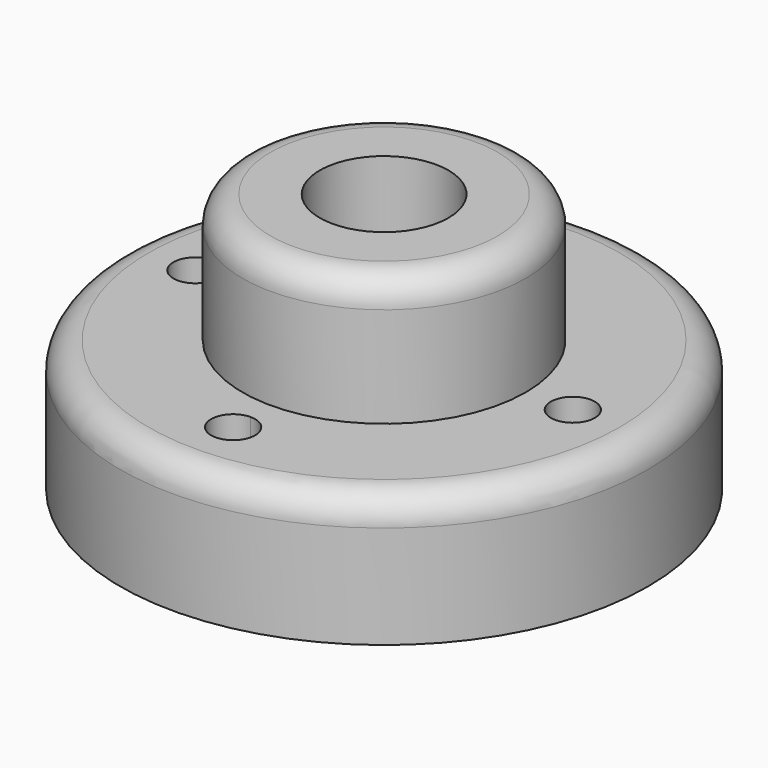
from build123d import *

# Parameters (mm, degrees)
F0_R     = 30
F0_R_2   = 16.1
F1_DEPTH = 14.9
F2_DEPTH = 29.5
F3_R     = 3.2
F4_R     = 3.2
F5_R     = 2.5
F6_DEPTH = 100
F7_R     = 7.315
F8_DEPTH = 100


with BuildPart() as f1:
    # F0 (on Top) → F1 (new body)
    with BuildSketch(Plane.XY):
        Circle(F0_R)
        Circle(F0_R_2, mode=Mode.SUBTRACT)
    extrude(amount=F1_DEPTH)

    # F0 (on Top) → F2 (join)
    with BuildSketch(Plane.XY):
        Circle(F0_R_2)
    extrude(amount=F2_DEPTH)

    # F3
    f3_edges = [f1.edges().sort_by_distance(p)[0] for p in [
        (-30, 0, 14.9),
    ]]
    fillet(f3_edges, radius=F3_R)

    # F4
    f4_edges = [f1.edges().sort_by_distance(p)[0] for p in [
        (-16.1, 0, 29.5),
    ]]
    fillet(f4_edges, radius=F4_R)

    # F5 (on face) → F6 (cut)
    with BuildSketch(Plane.XY.offset(14.9)):
        with Locations((0, 21.45)):
            Circle(F5_R)
        with BuildLine():
            ThreePointArc((23.95, 0), (21.45, 2.5), (18.95, 0))
            ThreePointArc((18.95, 0), (21.45, -2.5), (23.95, 0))
        make_face()
        with BuildLine():
            ThreePointArc((2.5, -21.45), (1.767766953, -19.682233047), (0, -18.95))
            ThreePointArc((0, -18.95), (-2.5, -21.45), (0, -23.95))
            ThreePointArc((0, -23.95), (1.767766953, -23.217766953), (2.5, -21.45))
        make_face()
        with Locations((-21.45, 0)):
            Circle(F5_R)
    extrude(amount=-F6_DEPTH, mode=Mode.SUBTRACT)

    # F7 (on face) → F8 (cut)
    with BuildSketch(Plane.XY.offset(29.5)):
        Circle(F7_R)
    extrude(amount=-F8_DEPTH, mode=Mode.SUBTRACT)


solid = f1.part
